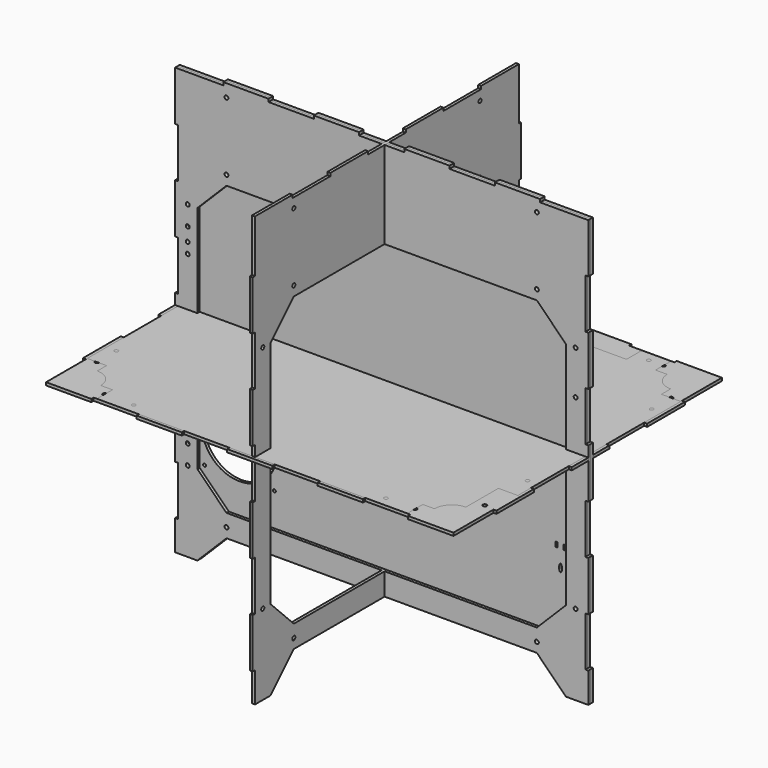
from build123d import *

# Parameters (mm, degrees)
F1_R     = 2
F2_DEPTH = 3
F3_R     = 2
F4_DEPTH = 3
F3_R_2   = 1.5
F3_R_3   = 39
F3_W     = 2
F3_H     = 5
F5_DEPTH = 3
F6_R     = 2
F7_DEPTH = 3
F8_R     = 2
F9_DEPTH = 3


# Not quite as in the source:
# - a feature names something its author has since deleted; it is built from what else it names


with BuildPart() as f2:
    # F1 (on Top) → F2 (new body)
    with BuildSketch(Plane.XY):
        Polygon((163.3333333333, -173), (210, -173), (210, -170), (210, -121.4285714286), (213, -121.4285714286), (213, -72.8571428571), (210, -72.8571428571), (210, -24.2857142857), (213, -24.2857142857), (213, 24.2857142857), (210, 24.2857142857), (210, 72.8571428571), (213, 72.8571428571), (213, 121.4285714286), (210, 121.4285714286), (210, 170), (210, 173), (163.3333333333, 173), (163.3333333333, 170), (116.6666666667, 170), (116.6666666667, 173), (70, 173), (70, 170), (23.3333333333, 170), (23.3333333333, 173), (-23.3333333333, 173), (-23.3333333333, 170), (-70, 170), (-70, 173), (-116.6666666667, 173), (-116.6666666667, 170), (-163.3333333333, 170), (-163.3333333333, 173), (-210, 173), (-210, 170), (-210, 121.4285714286), (-213, 121.4285714286), (-213, 72.8571428571), (-210, 72.8571428571), (-210, 24.2857142857), (-213, 24.2857142857), (-213, -24.2857142857), (-210, -24.2857142857), (-210, -72.8571428571), (-213, -72.8571428571), (-213, -121.4285714286), (-210, -121.4285714286), (-210, -170), (-210, -173), (-163.3333333333, -173), (-163.3333333333, -170), (-116.6666666667, -170), (-116.6666666667, -173), (-70, -173), (-70, -170), (-23.3333333333, -170), (-23.3333333333, -173), (23.3333333333, -173), (23.3333333333, -170), (70, -170), (70, -173), (116.6666666667, -173), (116.6666666667, -170), (163.3333333333, -170), align=None)
        with Locations((-160, -160)):
            Circle(F1_R, mode=Mode.SUBTRACT)
        with Locations((-200, -120)):
            Circle(F1_R, mode=Mode.SUBTRACT)
        with Locations((160, -160)):
            Circle(F1_R, mode=Mode.SUBTRACT)
        with Locations((200, -120)):
            Circle(F1_R, mode=Mode.SUBTRACT)
        with Locations((-200, 120)):
            Circle(F1_R, mode=Mode.SUBTRACT)
        with Locations((-160, 160)):
            Circle(F1_R, mode=Mode.SUBTRACT)
        Polygon((190, -120), (160, -150), (-160, -150), (-190, -120), (-190, 120), (-160, 150), (160, 150), (190, 120), align=None, mode=Mode.SUBTRACT)
        with Locations((200, 120)):
            Circle(F1_R, mode=Mode.SUBTRACT)
        with Locations((160, 160)):
            Circle(F1_R, mode=Mode.SUBTRACT)
    extrude(amount=F2_DEPTH)


with BuildPart() as f4:
    # F3 (on Front) → F4 (new body)
    with BuildSketch(Plane.XZ):
        Polygon((190, -221.5), (213, -221.5), (213, -190.3888888889), (210, -190.3888888889), (210, -139.2777777778), (213, -139.2777777778), (213, -88.1666666667), (210, -88.1666666667), (210, -37.0555555556), (213, -37.0555555556), (213, 14.0555555556), (210, 14.0555555556), (210, 65.1666666667), (213, 65.1666666667), (213, 116.2777777778), (210, 116.2777777778), (210, 167.3888888889), (213, 167.3888888889), (213, 218.5), (210, 218.5), (163.3333333333, 218.5), (163.3333333333, 221.5), (116.6666666667, 221.5), (116.6666666667, 218.5), (70, 218.5), (70, 221.5), (23.3333333333, 221.5), (23.3333333333, 218.5), (-23.3333333333, 218.5), (-23.3333333333, 221.5), (-70, 221.5), (-70, 218.5), (-116.6666666667, 218.5), (-116.6666666667, 221.5), (-163.3333333333, 221.5), (-163.3333333333, 218.5), (-210, 218.5), (-213, 218.5), (-213, 167.3888888889), (-210, 167.3888888889), (-210, 116.2777777778), (-213, 116.2777777778), (-213, 65.1666666667), (-210, 65.1666666667), (-210, 14.0555555556), (-213, 14.0555555556), (-213, -37.0555555556), (-210, -37.0555555556), (-210, -88.1666666667), (-213, -88.1666666667), (-213, -139.2777777778), (-210, -139.2777777778), (-210, -190.3888888889), (-213, -190.3888888889), (-213, -221.5), (-190, -221.5), (-160, -191.5), (160, -191.5), align=None)
        with Locations((-160, -181.5)):
            Circle(F3_R, mode=Mode.SUBTRACT)
        with Locations((-200, -138.5)):
            Circle(F3_R, mode=Mode.SUBTRACT)
        with Locations((-200, -118.5)):
            Circle(F3_R, mode=Mode.SUBTRACT)
        with Locations((-200, -104.5)):
            Circle(F3_R, mode=Mode.SUBTRACT)
        with Locations((160, -181.5)):
            Circle(F3_R, mode=Mode.SUBTRACT)
        with Locations((200, -138.5)):
            Circle(F3_R, mode=Mode.SUBTRACT)
        Polygon((-160, 128.5), (160, 128.5), (190, 98.5), (190, -138.5), (160, -168.5), (-160, -168.5), (-190, -138.5), (-190, 98.5), align=None, mode=Mode.SUBTRACT)
        with Locations((-200, 53.5)):
            Circle(F3_R, mode=Mode.SUBTRACT)
        with Locations((-200, 64.5)):
            Circle(F3_R, mode=Mode.SUBTRACT)
        with Locations((-200, 78.5)):
            Circle(F3_R, mode=Mode.SUBTRACT)
        with Locations((-200, 98.5)):
            Circle(F3_R, mode=Mode.SUBTRACT)
        with Locations((-160, 138.5)):
            Circle(F3_R, mode=Mode.SUBTRACT)
        with Locations((-160, 208.5)):
            Circle(F3_R, mode=Mode.SUBTRACT)
        with Locations((-140, 208.5)):
            Circle(F3_R, mode=Mode.SUBTRACT)
        with Locations((-126, 208.5)):
            Circle(F3_R, mode=Mode.SUBTRACT)
        with Locations((200, 53.5)):
            Circle(F3_R, mode=Mode.SUBTRACT)
        with Locations((200, 98.5)):
            Circle(F3_R, mode=Mode.SUBTRACT)
        with Locations((160, 138.5)):
            Circle(F3_R, mode=Mode.SUBTRACT)
        with Locations((126, 208.5)):
            Circle(F3_R, mode=Mode.SUBTRACT)
        with Locations((140, 208.5)):
            Circle(F3_R, mode=Mode.SUBTRACT)
        with Locations((160, 208.5)):
            Circle(F3_R, mode=Mode.SUBTRACT)
        with Locations((-140, 208.5)):
            Circle(F3_R)
        with Locations((-126, 208.5)):
            Circle(F3_R)
        with Locations((126, 208.5)):
            Circle(F3_R)
        with Locations((140, 208.5)):
            Circle(F3_R)
    extrude(amount=F4_DEPTH)


with BuildPart() as f5:
    # F3 (on Front) → F5 (new body)
    with BuildSketch(Plane.XZ):
        Polygon((190, -221.5), (213, -221.5), (213, -190.3888888889), (210, -190.3888888889), (210, -139.2777777778), (213, -139.2777777778), (213, -88.1666666667), (210, -88.1666666667), (210, -37.0555555556), (213, -37.0555555556), (213, 14.0555555556), (210, 14.0555555556), (210, 65.1666666667), (213, 65.1666666667), (213, 116.2777777778), (210, 116.2777777778), (210, 167.3888888889), (213, 167.3888888889), (213, 218.5), (210, 218.5), (163.3333333333, 218.5), (163.3333333333, 221.5), (116.6666666667, 221.5), (116.6666666667, 218.5), (70, 218.5), (70, 221.5), (23.3333333333, 221.5), (23.3333333333, 218.5), (-23.3333333333, 218.5), (-23.3333333333, 221.5), (-70, 221.5), (-70, 218.5), (-116.6666666667, 218.5), (-116.6666666667, 221.5), (-163.3333333333, 221.5), (-163.3333333333, 218.5), (-210, 218.5), (-213, 218.5), (-213, 167.3888888889), (-210, 167.3888888889), (-210, 116.2777777778), (-213, 116.2777777778), (-213, 65.1666666667), (-210, 65.1666666667), (-210, 14.0555555556), (-213, 14.0555555556), (-213, -37.0555555556), (-210, -37.0555555556), (-210, -88.1666666667), (-213, -88.1666666667), (-213, -139.2777777778), (-210, -139.2777777778), (-210, -190.3888888889), (-213, -190.3888888889), (-213, -221.5), (-190, -221.5), (-160, -191.5), (160, -191.5), align=None)
        with Locations((-160, -181.5)):
            Circle(F3_R, mode=Mode.SUBTRACT)
        with Locations((-200, -138.5)):
            Circle(F3_R, mode=Mode.SUBTRACT)
        with Locations((-200, -118.5)):
            Circle(F3_R, mode=Mode.SUBTRACT)
        with Locations((-200, -104.5)):
            Circle(F3_R, mode=Mode.SUBTRACT)
        with Locations((160, -181.5)):
            Circle(F3_R, mode=Mode.SUBTRACT)
        with Locations((200, -138.5)):
            Circle(F3_R, mode=Mode.SUBTRACT)
        Polygon((-160, 128.5), (160, 128.5), (190, 98.5), (190, -138.5), (160, -168.5), (-160, -168.5), (-190, -138.5), (-190, 98.5), align=None, mode=Mode.SUBTRACT)
        with Locations((-200, 53.5)):
            Circle(F3_R, mode=Mode.SUBTRACT)
        with Locations((-200, 64.5)):
            Circle(F3_R, mode=Mode.SUBTRACT)
        with Locations((-200, 78.5)):
            Circle(F3_R, mode=Mode.SUBTRACT)
        with Locations((-200, 98.5)):
            Circle(F3_R, mode=Mode.SUBTRACT)
        with Locations((-160, 138.5)):
            Circle(F3_R, mode=Mode.SUBTRACT)
        with Locations((-160, 208.5)):
            Circle(F3_R, mode=Mode.SUBTRACT)
        with Locations((-140, 208.5)):
            Circle(F3_R, mode=Mode.SUBTRACT)
        with Locations((-126, 208.5)):
            Circle(F3_R, mode=Mode.SUBTRACT)
        with Locations((200, 53.5)):
            Circle(F3_R, mode=Mode.SUBTRACT)
        with Locations((200, 98.5)):
            Circle(F3_R, mode=Mode.SUBTRACT)
        with Locations((160, 138.5)):
            Circle(F3_R, mode=Mode.SUBTRACT)
        with Locations((126, 208.5)):
            Circle(F3_R, mode=Mode.SUBTRACT)
        with Locations((140, 208.5)):
            Circle(F3_R, mode=Mode.SUBTRACT)
        with Locations((160, 208.5)):
            Circle(F3_R, mode=Mode.SUBTRACT)
        Polygon((190, 98.5), (160, 128.5), (-160, 128.5), (-190, 98.5), (-190, -138.5), (-160, -168.5), (160, -168.5), (190, -138.5), align=None)
        with Locations((-185, -134.5)):
            Circle(F3_R_2, mode=Mode.SUBTRACT)
        with Locations((-113, -134.5)):
            Circle(F3_R_2, mode=Mode.SUBTRACT)
        with Locations((-185, -62.5)):
            Circle(F3_R_2, mode=Mode.SUBTRACT)
        with Locations((-149, -98.5)):
            Circle(F3_R_3, mode=Mode.SUBTRACT)
        with Locations((-113, -62.5)):
            Circle(F3_R_2, mode=Mode.SUBTRACT)
        with BuildLine():
            add(Edge.make_bspline(
                [(182, -112.5), (184.5980762114, -112.5), (183.2990381057, -106.5), (182, -100.5), (180.7009618943, -106.5), (179.4019237886, -112.5), (182, -112.5)],
                knots=[0, 0, 0, 2.0943951024, 2.0943951024, 4.1887902048, 4.1887902048, 6.2831853072, 6.2831853072, 6.2831853072], degree=2, weights=[1, 0.5, 1, 0.5, 1, 0.5, 1]))
        make_face(mode=Mode.SUBTRACT)
        with Locations((178, -88.5)):
            Rectangle(F3_W, F3_H, mode=Mode.SUBTRACT)
        with Locations((186, -88.5)):
            Rectangle(F3_W, F3_H, mode=Mode.SUBTRACT)
        with BuildLine():
            Line((160, -15), (160, -10))
            ThreePointArc((160, -10), (170, -20), (160, -30))
            Line((160, -30), (160, -25))
            ThreePointArc((160, -25), (155, -20), (160, -15))
        make_face(mode=Mode.SUBTRACT)
        with Locations((-200, 78.5)):
            Circle(F3_R)
        with Locations((-200, -104.5)):
            Circle(F3_R)
        with Locations((-200, -118.5)):
            Circle(F3_R)
        with BuildLine():
            ThreePointArc((160, -30), (170, -20), (160, -10))
            Line((160, -10), (160, -15))
            ThreePointArc((160, -15), (155, -20), (160, -25))
            Line((160, -25), (160, -30))
        make_face()
    extrude(amount=-F5_DEPTH)


with BuildPart() as f7:
    # F6 (on Right) → F7 (new body)
    with BuildSketch(Plane.YZ):
        Polygon((-170, -221.5), (-150, -221.5), (-120, -191.5), (120, -191.5), (150, -221.5), (170, -221.5), (170, -190.3888888889), (173, -190.3888888889), (173, -139.2777777778), (170, -139.2777777778), (170, -88.1666666667), (173, -88.1666666667), (173, -37.0555555556), (170, -37.0555555556), (170, 14.0555555556), (173, 14.0555555556), (173, 65.1666666667), (170, 65.1666666667), (170, 116.2777777778), (173, 116.2777777778), (173, 167.3888888889), (170, 167.3888888889), (170, 218.5), (170, 221.5), (121.4285714286, 221.5), (121.4285714286, 218.5), (72.8571428571, 218.5), (72.8571428571, 221.5), (24.2857142857, 221.5), (24.2857142857, 218.5), (-24.2857142857, 218.5), (-24.2857142857, 221.5), (-72.8571428571, 221.5), (-72.8571428571, 218.5), (-121.4285714286, 218.5), (-121.4285714286, 221.5), (-170, 221.5), (-170, 218.5), (-170, 167.3888888889), (-173, 167.3888888889), (-173, 116.2777777778), (-170, 116.2777777778), (-170, 65.1666666667), (-173, 65.1666666667), (-173, 14.0555555556), (-170, 14.0555555556), (-170, -37.0555555556), (-173, -37.0555555556), (-173, -88.1666666667), (-170, -88.1666666667), (-170, -139.2777777778), (-173, -139.2777777778), (-173, -190.3888888889), (-170, -190.3888888889), align=None)
        with Locations((-120, -181.5)):
            Circle(F6_R, mode=Mode.SUBTRACT)
        with Locations((-160, -138.5)):
            Circle(F6_R, mode=Mode.SUBTRACT)
        with Locations((120, -181.5)):
            Circle(F6_R, mode=Mode.SUBTRACT)
        with Locations((160, -138.5)):
            Circle(F6_R, mode=Mode.SUBTRACT)
        with Locations((160, -118.5)):
            Circle(F6_R, mode=Mode.SUBTRACT)
        Polygon((-150, 98.5), (-120, 128.5), (120, 128.5), (150, 98.5), (150, -138.5), (120, -168.5), (-120, -168.5), (-150, -138.5), align=None, mode=Mode.SUBTRACT)
        with Locations((160, -104.5)):
            Circle(F6_R, mode=Mode.SUBTRACT)
        with Locations((-160, 98.5)):
            Circle(F6_R, mode=Mode.SUBTRACT)
        with Locations((-120, 138.5)):
            Circle(F6_R, mode=Mode.SUBTRACT)
        with Locations((-120, 208.5)):
            Circle(F6_R, mode=Mode.SUBTRACT)
        with Locations((160, 64.5)):
            Circle(F6_R, mode=Mode.SUBTRACT)
        with Locations((160, 78.5)):
            Circle(F6_R, mode=Mode.SUBTRACT)
        with Locations((160, 98.5)):
            Circle(F6_R, mode=Mode.SUBTRACT)
        with Locations((120, 138.5)):
            Circle(F6_R, mode=Mode.SUBTRACT)
        with Locations((120, 208.5)):
            Circle(F6_R, mode=Mode.SUBTRACT)
    extrude(amount=F7_DEPTH)


with BuildPart() as f9:
    # F8 (on Top) → F9 (new body)
    with BuildSketch(Plane.XY):
        with BuildLine():
            Line((160, -150), (172, -150))
            ThreePointArc((172, -150), (177.2720779386, -137.2720779386), (190, -132))
            Line((190, -132), (190, -90))
            Line((190, -90), (210, -90))
            Line((210, -90), (210, 120))
            Line((210, 120), (190, 120))
            Line((190, 120), (190, 132))
            ThreePointArc((190, 132), (177.2720779386, 137.2720779386), (172, 150))
            Line((172, 150), (160, 150))
            Line((160, 150), (160, 170))
            Line((160, 170), (130, 170))
            Line((130, 170), (130, 150))
            Line((130, 150), (37.5, 150))
            Line((37.5, 150), (37.5, 147))
            Line((37.5, 147), (24.5, 147))
            Line((24.5, 147), (24.5, 107))
            Line((24.5, 107), (-24.5, 107))
            Line((-24.5, 107), (-24.5, 147))
            Line((-24.5, 147), (-37.5, 147))
            Line((-37.5, 147), (-37.5, 150))
            Line((-37.5, 150), (-130, 150))
            Line((-130, 150), (-130, 170))
            Line((-130, 170), (-160, 170))
            Line((-160, 170), (-160, 150))
            Line((-160, 150), (-172, 150))
            ThreePointArc((-172, 150), (-177.2720779386, 137.2720779386), (-190, 132))
            Line((-190, 132), (-190, 90))
            Line((-190, 90), (-210, 90))
            Line((-210, 90), (-210, -120))
            Line((-210, -120), (-190, -120))
            Line((-190, -120), (-190, -132))
            ThreePointArc((-190, -132), (-177.2720779386, -137.2720779386), (-172, -150))
            Line((-172, -150), (-160, -150))
            Line((-160, -150), (-160, -170))
            Line((-160, -170), (160, -170))
            Line((160, -170), (160, -150))
        make_face()
        with Locations((-130, -160)):
            Circle(F8_R, mode=Mode.SUBTRACT)
        with Locations((-200, -95)):
            Circle(F8_R, mode=Mode.SUBTRACT)
        with Locations((130, -160)):
            Circle(F8_R, mode=Mode.SUBTRACT)
        with Locations((200, -65)):
            Circle(F8_R, mode=Mode.SUBTRACT)
        with Locations((-200, 65)):
            Circle(F8_R, mode=Mode.SUBTRACT)
        with Locations((-145, 160)):
            Circle(F8_R, mode=Mode.SUBTRACT)
        with Locations((200, 95)):
            Circle(F8_R, mode=Mode.SUBTRACT)
        with Locations((145, 160)):
            Circle(F8_R, mode=Mode.SUBTRACT)
    extrude(amount=F9_DEPTH)


solid = Compound([f2.part, f4.part, f5.part, f7.part, f9.part])
